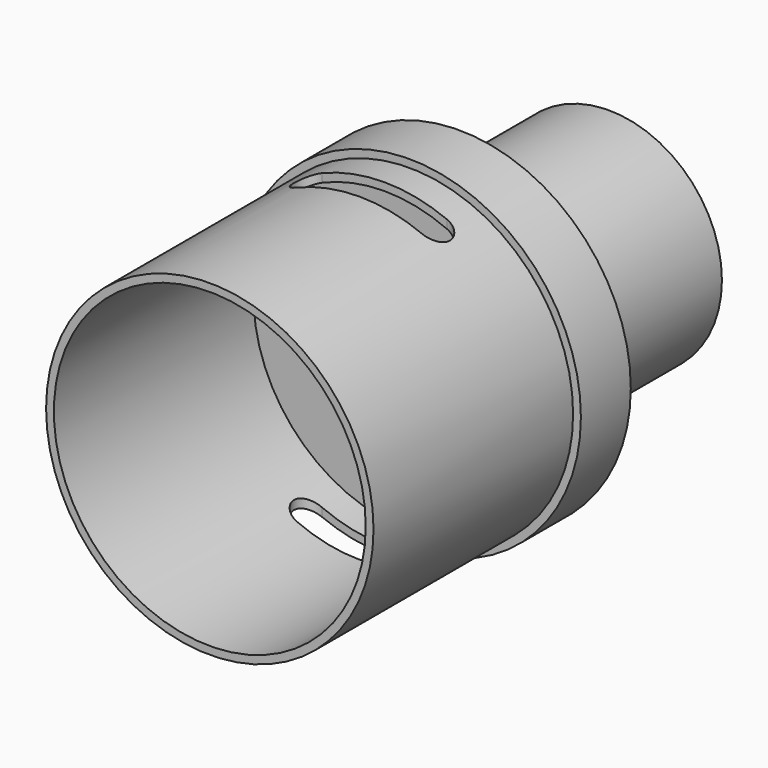
from build123d import *

# Parameters (mm, degrees)
F0_R     = 4.6
F0_R_2   = 3.965
F1_DEPTH = 7.62
F0_R_3   = 6.985
F0_R_4   = 6.35
F2_DEPTH = 2.54
F3_DEPTH = 12.7
F5_R     = 6.985
F5_R_2   = 6.6675
F6_DEPTH = 10.16
F7_DEPTH = 6.82625


# Not quite as in the source:
# - a feature names something its author has since deleted; it is built from what else it names


with BuildPart() as f1:
    # F0 (on Front) → F1 (new body)
    with BuildSketch(Plane.XZ):
        Circle(F0_R)
        Circle(F0_R_2, mode=Mode.SUBTRACT)
    extrude(amount=-F1_DEPTH)

    # F0 (on Front) → F2 (join)
    with BuildSketch(Plane.XZ):
        Circle(F0_R_3)
        Circle(F0_R_4, mode=Mode.SUBTRACT)
        Circle(F0_R_4)
        Circle(F0_R, mode=Mode.SUBTRACT)
        Circle(F0_R)
        Circle(F0_R_2, mode=Mode.SUBTRACT)
    extrude(amount=F2_DEPTH)

    # F0 (on Front) → F3 (join)
    with BuildSketch(Plane.XZ):
        Circle(F0_R_3)
        Circle(F0_R_4, mode=Mode.SUBTRACT)
    extrude(amount=F3_DEPTH)

    # F5 (on face) → F6 (cut)
    with BuildSketch(Plane.XZ.offset(12.7)):
        Circle(F5_R)
        Circle(F5_R_2, mode=Mode.SUBTRACT)
    extrude(amount=-F6_DEPTH, mode=Mode.SUBTRACT)

    # F4 (on Top) → F7 (cut, symmetric)
    with BuildSketch(Plane.XY):
        with BuildLine():
            Line((2.54, -3.81), (0, -3.81))
            Line((0, -3.81), (-2.54, -3.81))
            ThreePointArc((-2.54, -3.81), (-3.175, -4.445), (-2.54, -5.08))
            Line((-2.54, -5.08), (0, -5.08))
            Line((0, -5.08), (2.54, -5.08))
            ThreePointArc((2.54, -5.08), (3.175, -4.445), (2.54, -3.81))
        make_face()
    extrude(amount=F7_DEPTH, both=True, mode=Mode.SUBTRACT)


solid = f1.part
